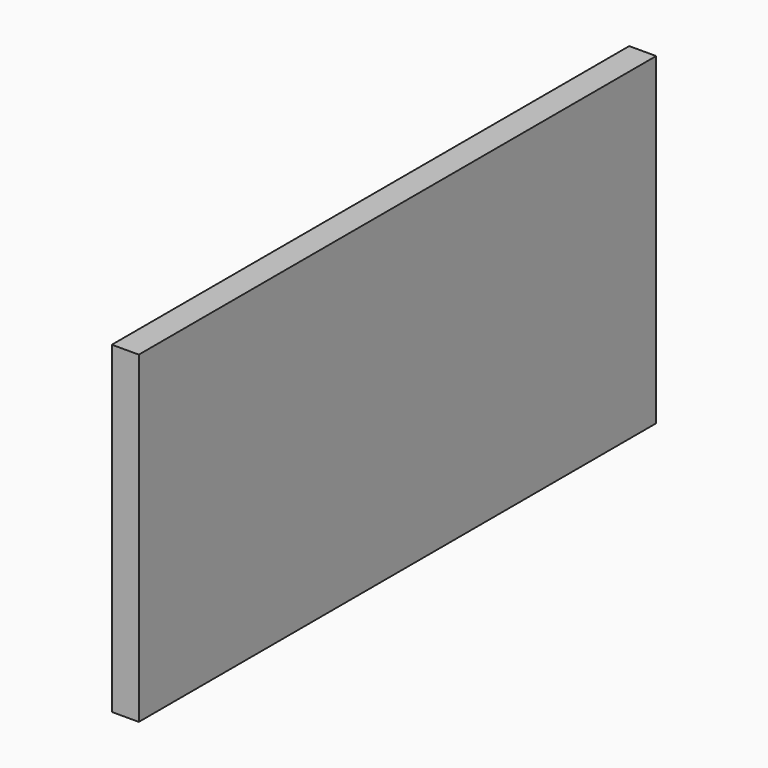
from build123d import *

# Parameters (mm, degrees)
F0_W     = 152.4
F0_H     = 76.2
F1_DEPTH = 6.35


# Not quite as in the source:
# - a length typed as a fraction of an inch, garbled in the dataset ("3 / 203.2 mm" for 3/8 in), is restored


with BuildPart() as f1:
    # F0 (on Right) → F1 (new body)
    with BuildSketch(Plane.YZ):
        Rectangle(F0_W, F0_H)
    extrude(amount=F1_DEPTH)


solid = f1.part
